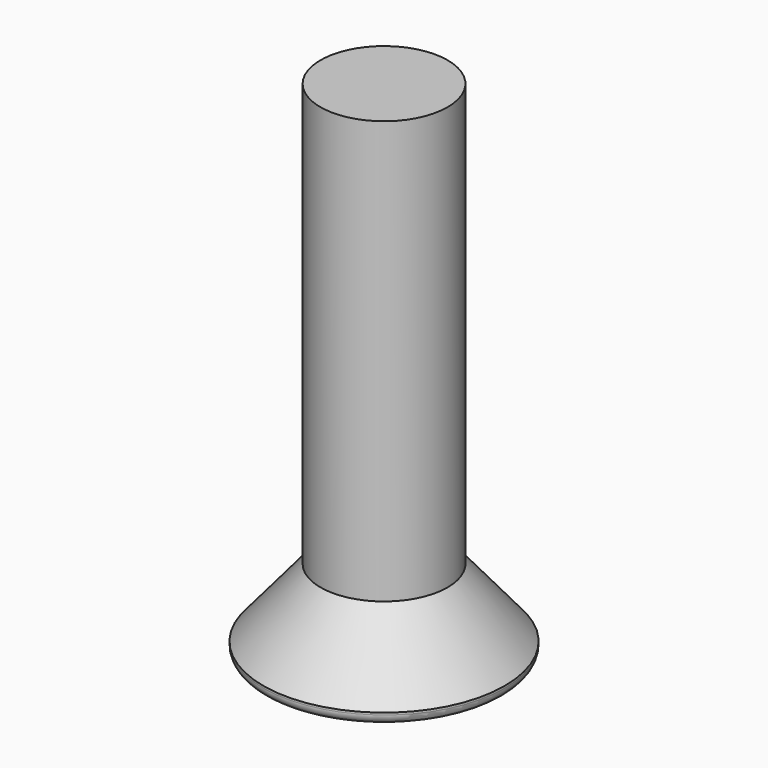
from build123d import *

# Parameters (mm, degrees)
F0_R        = 6
F0_R_2      = 3.16
F1_DEPTH    = 4
F2_DEPTH    = 25
F3_S5_R     = 3.16
F3_T6_DEPTH = 10
F4_R        = 0.5


# Not quite as in the source:
# - a fillet or chamfer that OpenCascade refuses, or shapes differently, is made with other operations: its cross-section is extruded or revolved along the edge and cut away or added


with BuildPart() as f1:
    # F0 (on Top) → F1 (new body)
    with BuildSketch(Plane.XY):
        Circle(F0_R)
        Circle(F0_R_2, mode=Mode.SUBTRACT)
    extrude(amount=F1_DEPTH)

    # F0 (on Top) → F2 (join)
    with BuildSketch(Plane.XY):
        Circle(F0_R_2)
    extrude(amount=F2_DEPTH)

    # F3: chamfer of 2.85 x 3.3964977389 on 1 edges, made by hand


with BuildPart() as f3_tool2:
    # F3_s3 → F3_t4 (revolve)
    with BuildSketch(Plane.XZ):
        Polygon((6, 0.6035022611), (3.15, 4), (6, 4), align=None)
    revolve(axis=Axis((0, 0, 4), (0, 0, 1)))

    # F3_s5 → F3_t6 (cut, symmetric)
    with BuildSketch(Plane.XY.offset(2.3)):
        Circle(F3_S5_R)
    extrude(amount=F3_T6_DEPTH, both=True, mode=Mode.SUBTRACT)


with BuildPart() as f1_1:
    add(f1.part)

    # F3_t1: cut F3_tool2
    add(f3_tool2.part, mode=Mode.SUBTRACT)

    # F4
    f4_edges = [f1_1.edges().sort_by_distance(p)[0] for p in [
        (-6, 0, 0),
    ]]
    fillet(f4_edges, radius=F4_R)


solid = f1_1.part
